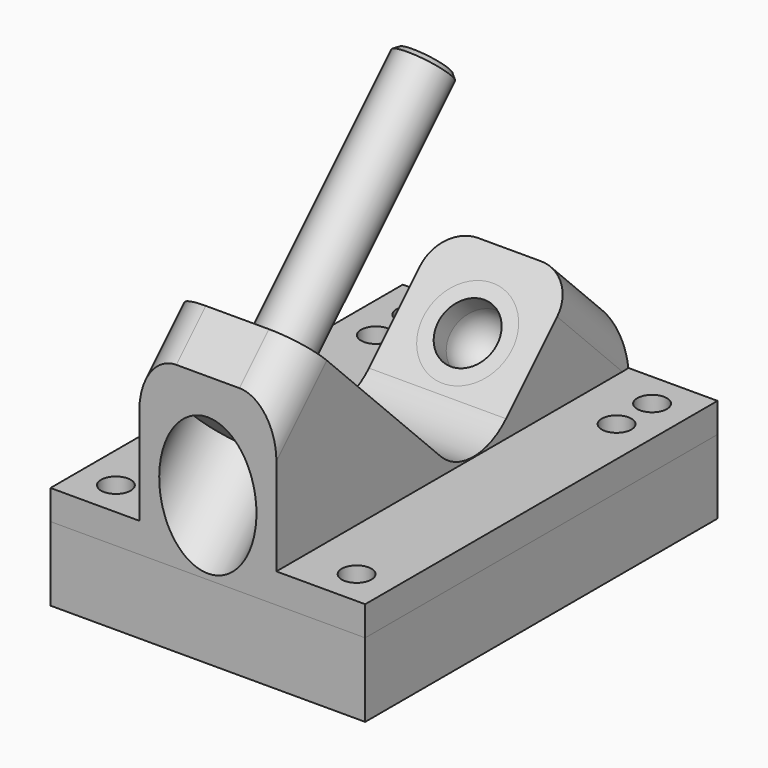
from build123d import *

# Parameters (mm, degrees)
F1_DEPTH  = 27.0002
F2_R      = 9.906
F3_W      = 75.565
F3_H      = 31.9504877579
F4_DEPTH  = 15.24
F5_R      = 2.54
F6_DEPTH  = 5.081
F8_R      = 6.35
F13_SIZE  = 0.762
F16_DEPTH = 12.7


with BuildPart() as f1:
    # F0 (on Right) → F1 (new body)
    with BuildSketch(Plane.YZ):
        Polygon((0, 30.6972561211), (0, 0), (75.565, 0), (75.565, 12.7), (64.7048964237, 23.5601035763), (42.2542561211, 1.1094632736), (6.3332316368, 37.0304877579), align=None)
    extrude(amount=F1_DEPTH)

    # F2
    f2_edges = [f1.edges().sort_by_distance(p)[0] for p in [
        (13.5001, 42.254256, 1.109463),
    ]]
    fillet(f2_edges, radius=F2_R)

    # F3 (on face) → F4 (cut)
    with BuildSketch(Plane.YZ.offset(27.0002)):
        with Locations((37.7825, 21.0552438789)):
            Rectangle(F3_W, F3_H)
    extrude(amount=-F4_DEPTH, mode=Mode.SUBTRACT)

    # F5 (on face) → F6 (cut, through all)
    with BuildSketch(Plane.XY.offset(5.08)):
        with Locations((20.6502, 69.469)):
            Circle(F5_R)
        with Locations((20.6502, 61.849)):
            Circle(F5_R)
        with Locations((20.6502, 6.096)):
            Circle(F5_R)
    extrude(amount=-F6_DEPTH, mode=Mode.SUBTRACT)

    # F7: F1 across face


with BuildPart() as f1_1:
    add(f1.part)
    add(f1.part.mirror(Plane(origin=(0, 31.4297936493, 11.6265989231), x_dir=(0, 1, 0), z_dir=(-1, 0, 0))))

    # F8
    f8_edges = [f1_1.edges().sort_by_distance(p)[0] for p in [
        (-11.7602, 70.134948, 18.130052),
        (-11.7602, 3.166616, 33.863872),
        (11.7602, 3.166616, 33.863872),
        (11.7602, 70.134948, 18.130052),
    ]]
    fillet(f8_edges, radius=F8_R)

    # F9 (on Right) → F10 (revolve, cut)
    with BuildSketch(Plane.YZ):
        Polygon((-6.3683719395, 6.3683719395), (15.3134877579, 28.0502316368), (11.9458917125, 31.4178276822), (5.2106996217, 24.6826355914), (2.6782673955, 27.2150678175), (-12.268400211, 12.268400211), align=None)
    revolve(axis=Axis((0, 22.0486798487, 34.7854237276), (0, 0.7071067812, 0.7071067812)), mode=Mode.SUBTRACT)

    # F14 (on Right) → F15 (revolve, cut)
    with BuildSketch(Plane.YZ):
        Polygon((61.1127939753, 19.9680011278), (55.7246403027, 14.5798474552), (64.7048964237, 5.5995913341), (70.0930500964, 10.9877450068), align=None)
    revolve(axis=Axis((0, 60.2147683632, 10.0897193947), (0, -0.7071067812, 0.7071067812)), mode=Mode.SUBTRACT)


with BuildPart() as f12:
    # F11 (on Right) → F12 (revolve)
    with BuildSketch(Plane.YZ):
        Polygon((11.9458917125, 31.4178276822), (5.2106996217, 24.6826355914), (2.9656355914, 26.9276996217), (1.1695843672, 25.1316483974), (6.7822444428, 19.5189883218), (46.7443841816, 59.4811280605), (43.3767881362, 62.8487241059), align=None)
    revolve(axis=Axis((0, 26.7633143122, 39.5000581912), (0, 0.7071067812, 0.7071067812)))

    # F13
    f13_edges = [f12.edges().sort_by_distance(p)[0] for p in [
        (0, 50.11198, 56.113532),
    ]]
    chamfer(f13_edges, length=F13_SIZE)


with BuildPart() as f16:
    # F16 (new): a face of the model
    f16_faces = [f1_1.part.faces().sort_by_distance(p)[0] for p in [
        (0, 37.5360763609, 0),
    ]]
    extrude(f16_faces, amount=F16_DEPTH)


with BuildPart() as f18:
    # F17 (on Right) → F18 (revolve)
    with BuildSketch(Plane.YZ):
        with BuildLine():
            Line((59.3167427511, 18.1719499036), (62.0108195874, 15.4778730673))
            ThreePointArc((62.0108195874, 15.4778730673), (63.498717139, 11.8857706189), (62.0108195874, 8.2936681704))
            Line((62.0108195874, 8.2936681704), (64.7048964237, 5.5995913341))
            Line((64.7048964237, 5.5995913341), (70.0930500964, 10.9877450068))
            Line((70.0930500964, 10.9877450068), (61.1127939753, 19.9680011278))
            Line((61.1127939753, 19.9680011278), (59.3167427511, 18.1719499036))
        make_face()
    revolve(axis=Axis((0, 60.2147683632, 10.0897193947), (0, -0.7071067812, 0.7071067812)))


solid = Compound([f1_1.part, f12.part, f16.part, f18.part])
